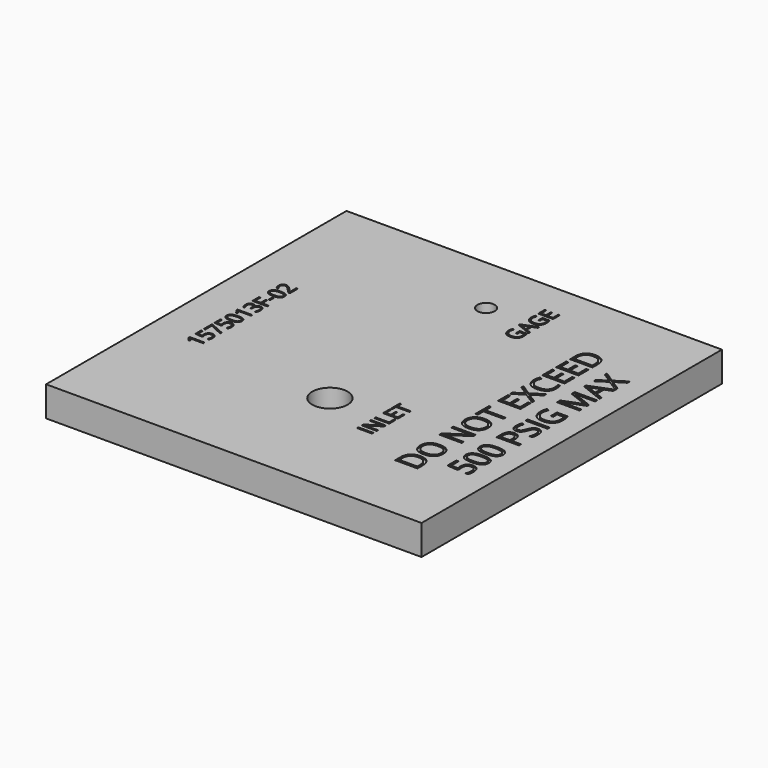
from build123d import *

# Parameters (mm, degrees)
F0_W           = 79.375
F0_H           = 79.375
F1_DEPTH       = 6.35
F2_R           = 1.8288
F2_R_2         = 3.7465
F3_DEPTH       = 25.4
F2_TEXT_SIZE   = 4.4097222222
F2_TEXT_SIZE_2 = 6.6145833333
F4_DEPTH       = 0.254


# Not quite as in the source:
# - Text() gives the source's letters only with a copy of the font that has no kerning and outlines rounded to 1/6400 em; it was checked with that copy


with BuildPart() as f1:
    # F0 (on Top) → F1 (new body)
    with BuildSketch(Plane.XY):
        Rectangle(F0_W, F0_H)
    extrude(amount=F1_DEPTH)

    # F2 (on face) → F3 (cut)
    with BuildSketch(Plane.XY.offset(6.35)):
        with Locations((0, 26.9875)):
            Circle(F2_R)
        with Locations((0, -14.2875)):
            Circle(F2_R_2)
    extrude(amount=-F3_DEPTH, mode=Mode.SUBTRACT)

    # F2 (on face) → F4 (cut)
    with BuildSketch(Plane.XY.offset(6.35)):
        with Locations((0, 26.9875)):
            Circle(F2_R)
        with Locations((0, -14.2875)):
            Circle(F2_R_2)
        with Locations(Location((13.335, -20.2771430122), (0, 0, 90))):
            Text('INLET', F2_TEXT_SIZE, font='Open Sans', text_align=(TextAlign.LEFT, TextAlign.BOTTOM))
        with Locations(Location((11.1125, 21.1453070747), (0, 0, 90))):
            Text('GAGE', F2_TEXT_SIZE, font='Open Sans', text_align=(TextAlign.LEFT, TextAlign.BOTTOM))
        with Locations(Location((26.9875, -25.5410766602), (0, 0, 90))):
            Text('DO NOT EXCEED', F2_TEXT_SIZE_2, font='Open Sans', text_align=(TextAlign.LEFT, TextAlign.BOTTOM))
        with Locations(Location((34.925, -21.7165039063), (0, 0, 90))):
            Text('500 PSIG MAX', F2_TEXT_SIZE_2, font='Open Sans', text_align=(TextAlign.LEFT, TextAlign.BOTTOM))
        with Locations(Location((-28.575, -13.2171088325), (0, 0, 90))):
            Text('1575013F-02', F2_TEXT_SIZE, font='Open Sans', text_align=(TextAlign.LEFT, TextAlign.BOTTOM))
    extrude(amount=-F4_DEPTH, mode=Mode.SUBTRACT)


solid = f1.part
